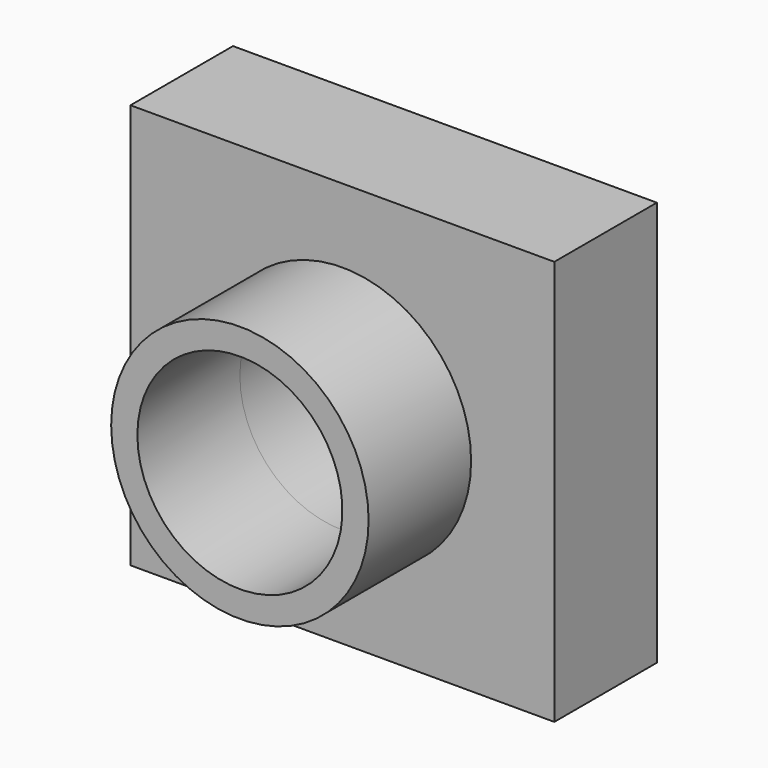
from build123d import *

# Parameters (mm, degrees)
F0_W     = 82.6933681965
F0_H     = 79.0255218744
F2_DEPTH = 25
F1_R     = 25.1134324312
F3_DEPTH = 25
F5_D     = 40
F5_2_D   = 40
F5_3_D   = 40


with BuildPart() as f2:
    # F0 (on Front) → F2 (new body)
    with BuildSketch(Plane.XZ):
        Rectangle(F0_W, F0_H)
    extrude(amount=F2_DEPTH)

    # F5 (through all)
    with Locations(Plane(origin=(0, 0, 0), x_dir=(1, 0, 0), z_dir=(0, 1, 0))):
        with Locations((0, 0)):
            Hole(F5_D / 2)


with BuildPart() as f2b:
    # F1 (on Front) → F2, piece 2 (new body)
    with BuildSketch(Plane.XZ):
        Circle(F1_R)
    extrude(amount=F2_DEPTH)


with BuildPart() as f3:
    # F3 (new): a face of the model
    f3_faces = [f2b.part.faces().sort_by_distance(p)[0] for p in [
        (0, -25, 0),
    ]]
    extrude(f3_faces, amount=F3_DEPTH)

    # F5#3 (through all)
    with Locations(Plane(origin=(0, 0, 0), x_dir=(1, 0, 0), z_dir=(0, 1, 0))):
        with Locations((0, 0)):
            Hole(F5_3_D / 2)


with BuildPart() as f2b_1:
    add(f2b.part)

    # F5#2 (through all)
    with Locations(Plane(origin=(0, 0, 0), x_dir=(1, 0, 0), z_dir=(0, 1, 0))):
        with Locations((0, 0)):
            Hole(F5_2_D / 2)


solid = Compound([f2.part, f3.part, f2b_1.part])
